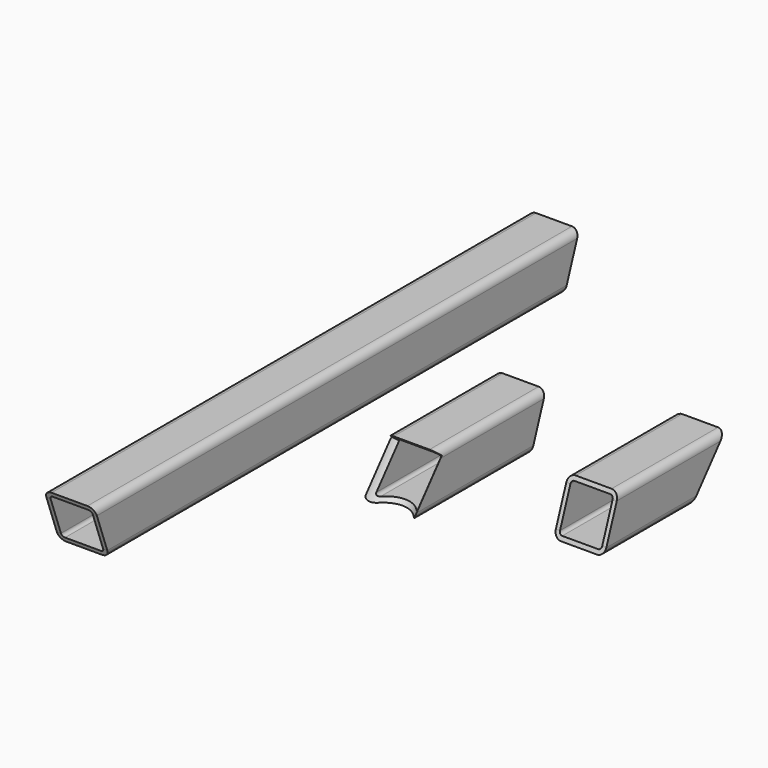
from build123d import *

# Parameters (mm, degrees)
F1_DEPTH  = 304.8
F3_DEPTH  = 101.6
F5_DEPTH  = 25.4
F7_DEPTH  = 25.4
F10_R     = 14.2875
F11_DEPTH = 40.64
F13_DEPTH = 76.2
F15_DEPTH = 25.4


with BuildPart() as f1:
    # F0 (on Front) → F1 (new body)
    with BuildSketch(Plane.XZ):
        with BuildLine():
            Line((-37.9424992715, 53.3812791109), (-55.9764980507, 53.3812791109))
            ThreePointArc((-55.9764980507, 53.3812791109), (-58.5807727574, 52.3025532072), (-59.6594986611, 49.6982785005))
            Line((-59.6594986611, 49.6982785005), (-59.6594986611, 31.6642797213))
            ThreePointArc((-59.6594986611, 31.6642797213), (-58.5807727574, 29.0600050146), (-55.9764980507, 27.9812791109))
            Line((-55.9764980507, 27.9812791109), (-37.9424992715, 27.9812791109))
            ThreePointArc((-37.9424992715, 27.9812791109), (-35.3382245648, 29.0600050146), (-34.2594986611, 31.6642797213))
            Line((-34.2594986611, 31.6642797213), (-34.2594986611, 49.6982785005))
            ThreePointArc((-34.2594986611, 49.6982785005), (-35.3382245648, 52.3025532072), (-37.9424992715, 53.3812791109))
        make_face()
        with BuildLine():
            ThreePointArc((-57.5766980507, 49.6982785005), (-57.108010322, 50.8297907718), (-55.9764980507, 51.2984785005))
            Line((-55.9764980507, 51.2984785005), (-37.9424992715, 51.2984785005))
            ThreePointArc((-37.9424992715, 51.2984785005), (-36.8109870002, 50.8297907718), (-36.3422992715, 49.6982785005))
            Line((-36.3422992715, 49.6982785005), (-36.3422992715, 31.6642797213))
            ThreePointArc((-36.3422992715, 31.6642797213), (-36.8109870002, 30.53276745), (-37.9424992715, 30.0640797213))
            Line((-37.9424992715, 30.0640797213), (-55.9764980507, 30.0640797213))
            ThreePointArc((-55.9764980507, 30.0640797213), (-57.108010322, 30.53276745), (-57.5766980507, 31.6642797213))
            Line((-57.5766980507, 31.6642797213), (-57.5766980507, 49.6982785005))
        make_face(mode=Mode.SUBTRACT)
    extrude(amount=F1_DEPTH)

    # F4 (on face) → F5 (cut, through all)
    with BuildSketch(Plane(origin=(-59.6594986611, 0, 0), x_dir=(0, -1, 0), z_dir=(-1, 0, 0))):
        Polygon((7.9043413554, 31.6642797213), (1.340502595, 49.6982785005), (0, 49.6982785005), (0, 31.6642797213), align=None)
        Polygon((1.340502595, 49.6982785005), (0, 53.3812791109), (0, 49.6982785005), align=None)
        Polygon((9.2448439504, 27.9812791109), (7.9043413554, 31.6642797213), (0, 31.6642797213), (0, 27.9812791109), align=None)
        Polygon((304.8, 53.3812791109), (303.459497405, 49.6982785005), (304.8, 49.6982785005), align=None)
        Polygon((304.8, 49.6982785005), (303.459497405, 49.6982785005), (296.8956586446, 31.6642797213), (304.8, 31.6642797213), align=None)
        Polygon((304.8, 31.6642797213), (296.8956586446, 31.6642797213), (295.5551560496, 27.9812791109), (304.8, 27.9812791109), align=None)
    extrude(amount=-F5_DEPTH, mode=Mode.SUBTRACT)


with BuildPart() as f3:
    # F2 (on Front) → F3 (new body)
    with BuildSketch(Plane.XZ):
        with BuildLine():
            Line((-54.7259064655, -23.0876084745), (-72.7599052448, -23.0876084745))
            ThreePointArc((-72.7599052448, -23.0876084745), (-75.3641799515, -24.1663343782), (-76.4429058552, -26.7706090849))
            Line((-76.4429058552, -26.7706090849), (-76.4429058552, -44.8046078641))
            ThreePointArc((-76.4429058552, -44.8046078641), (-75.3641799515, -47.4088825708), (-72.7599052448, -48.4876084745))
            Line((-72.7599052448, -48.4876084745), (-54.7259064655, -48.4876084745))
            ThreePointArc((-54.7259064655, -48.4876084745), (-52.1216317588, -47.4088825708), (-51.0429058552, -44.8046078641))
            Line((-51.0429058552, -44.8046078641), (-51.0429058552, -26.7706090849))
            ThreePointArc((-51.0429058552, -26.7706090849), (-52.1216317588, -24.1663343782), (-54.7259064655, -23.0876084745))
        make_face()
        with BuildLine():
            ThreePointArc((-74.3601052448, -26.7706090849), (-73.8914175161, -25.6390968136), (-72.7599052448, -25.1704090849))
            Line((-72.7599052448, -25.1704090849), (-54.7259064655, -25.1704090849))
            ThreePointArc((-54.7259064655, -25.1704090849), (-53.5943941943, -25.6390968136), (-53.1257064655, -26.7706090849))
            Line((-53.1257064655, -26.7706090849), (-53.1257064655, -44.8046078641))
            ThreePointArc((-53.1257064655, -44.8046078641), (-53.5943941943, -45.9361201354), (-54.7259064655, -46.4048078641))
            Line((-54.7259064655, -46.4048078641), (-72.7599052448, -46.4048078641))
            ThreePointArc((-72.7599052448, -46.4048078641), (-73.8914175161, -45.9361201354), (-74.3601052448, -44.8046078641))
            Line((-74.3601052448, -44.8046078641), (-74.3601052448, -26.7706090849))
        make_face(mode=Mode.SUBTRACT)
    extrude(amount=F3_DEPTH)

    # F6 (on face) → F7 (cut, through all)
    with BuildSketch(Plane(origin=(-76.4429058552, 0, 0), x_dir=(0, -1, 0), z_dir=(-1, 0, 0))):
        Polygon((1.340502595, -26.7706090849), (0, -26.7706090849), (0, -44.8046078641), (7.9043413554, -44.8046078641), align=None)
        Polygon((7.9043413554, -44.8046078641), (0, -44.8046078641), (0, -48.4876084745), (9.2448439504, -48.4876084745), align=None)
        Polygon((1.340502595, -26.7706090849), (0, -23.0876084745), (0, -26.7706090849), align=None)
        Polygon((80.2868693681, -23.0876084745), (83.3772738219, -26.7706090849), (101.6, -26.7706090849), (101.6, -23.0876084745), align=None)
        Polygon((101.6, -26.7706090849), (83.3772738219, -26.7706090849), (98.5095955462, -44.8046078641), (101.6, -44.8046078641), align=None)
        Polygon((101.6, -44.8046078641), (98.5095955462, -44.8046078641), (101.6, -48.4876084745), align=None)
    extrude(amount=-F7_DEPTH, mode=Mode.SUBTRACT)

    # F10 (on face) → F11 (cut)
    with BuildSketch(Plane(origin=(0, -65.8541589499, -78.4819305158), x_dir=(1, 0, 0), z_dir=(0, 0.6427876097, 0.7660444431))):
        with Locations((-63.7429058552, -40.1174512895)):
            Circle(F10_R)
    extrude(amount=F11_DEPTH, mode=Mode.SUBTRACT)


with BuildPart() as f13:
    # F12 (on Front) → F13 (new body)
    with BuildSketch(Plane.XZ):
        with BuildLine():
            Line((35.5612983663, -11.7608893991), (17.527299587, -11.7608893991))
            ThreePointArc((17.527299587, -11.7608893991), (14.9230248803, -12.8396153027), (13.8442989767, -15.4438900094))
            Line((13.8442989767, -15.4438900094), (13.8442989767, -33.4778887887))
            ThreePointArc((13.8442989767, -33.4778887887), (14.9230248803, -36.0821634954), (17.527299587, -37.1608893991))
            Line((17.527299587, -37.1608893991), (35.5612983663, -37.1608893991))
            ThreePointArc((35.5612983663, -37.1608893991), (38.165573073, -36.0821634954), (39.2442989767, -33.4778887887))
            Line((39.2442989767, -33.4778887887), (39.2442989767, -15.4438900094))
            ThreePointArc((39.2442989767, -15.4438900094), (38.165573073, -12.8396153027), (35.5612983663, -11.7608893991))
        make_face()
        with BuildLine():
            ThreePointArc((15.927099587, -15.4438900094), (16.3957873158, -14.3123777382), (17.527299587, -13.8436900094))
            Line((17.527299587, -13.8436900094), (35.5612983663, -13.8436900094))
            ThreePointArc((35.5612983663, -13.8436900094), (36.6928106376, -14.3123777382), (37.1614983663, -15.4438900094))
            Line((37.1614983663, -15.4438900094), (37.1614983663, -33.4778887887))
            ThreePointArc((37.1614983663, -33.4778887887), (36.6928106376, -34.6094010599), (35.5612983663, -35.0780887887))
            Line((35.5612983663, -35.0780887887), (17.527299587, -35.0780887887))
            ThreePointArc((17.527299587, -35.0780887887), (16.3957873158, -34.6094010599), (15.927099587, -33.4778887887))
            Line((15.927099587, -33.4778887887), (15.927099587, -15.4438900094))
        make_face(mode=Mode.SUBTRACT)
    extrude(amount=F13_DEPTH)

    # F14 (on face) → F15 (cut, through all)
    with BuildSketch(Plane.YZ.offset(39.2442989767)):
        Polygon((-76.2, -15.4438900094), (-68.2956586446, -15.4438900094), (-66.9551560496, -11.7608893991), (-76.2, -11.7608893991), align=None)
        Polygon((-74.859497405, -33.4778887887), (-68.2956586446, -15.4438900094), (-76.2, -15.4438900094), (-76.2, -33.4778887887), align=None)
        Polygon((-76.2, -37.1608893991), (-74.859497405, -33.4778887887), (-76.2, -33.4778887887), align=None)
        Polygon((0, -33.4778887887), (-18.2227261781, -33.4778887887), (-21.3131306319, -37.1608893991), (0, -37.1608893991), align=None)
        Polygon((0, -15.4438900094), (-3.0904044538, -15.4438900094), (-18.2227261781, -33.4778887887), (0, -33.4778887887), align=None)
        Polygon((0, -15.4438900094), (0, -11.7608893991), (-3.0904044538, -15.4438900094), align=None)
    extrude(amount=-F15_DEPTH, mode=Mode.SUBTRACT)


solid = Compound([f1.part, f3.part, f13.part])
